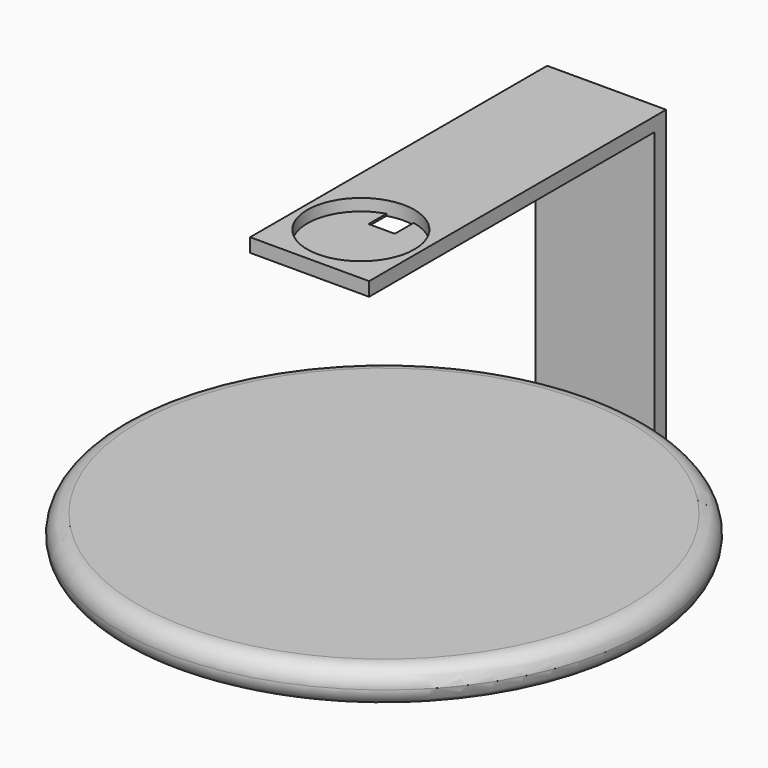
from build123d import *

# Parameters (mm, degrees)
F0_R      = 28.1709911247
F1_DEPTH  = 3.81
F2_R      = 1.90499
F4_DEPTH  = 31.75
F5_W      = 12.7
F5_H      = 1.4726919234
F6_DEPTH  = 38.1
F8_DEPTH  = 12.7
F9_R      = 5.715
F10_DEPTH = 1.27
F12_DEPTH = 25.4


# Not quite as in the source:
# - a fillet or chamfer is up to 0.001 mm smaller than in the source, because OpenCascade refuses the exact size


with BuildPart() as f1:
    # F0 (on Top) → F1 (new body)
    with BuildSketch(Plane.XY):
        Circle(F0_R)
    extrude(amount=F1_DEPTH)

    # F2 (radius 1.905 in the source; OpenCascade refuses exactly that, so slightly less here)
    f2_edges = [f1.edges().sort_by_distance(p)[0] for p in [
        (-28.170991, 0, 3.81),
        (-28.170991, 0, 0),
    ]]
    fillet(f2_edges, radius=F2_R)


with BuildPart() as f4:
    # F3 (on face) → F4 (new body)
    with BuildSketch(Plane(origin=(0, 0, 0), x_dir=(1, 0, 0), z_dir=(0, 0, -1))):
        Polygon((6.35, -28.1780194491), (0, -28.1780194491), (-6.35, -28.1780194491), (-6.35, -29.7020194491), (6.35, -29.7020194491), align=None)
    extrude(amount=-F4_DEPTH)

    # F5 (on face) → F6 (join)
    with BuildSketch(Plane.XZ.offset(-28.1780194491)):
        with Locations((0, 31.0136540383)):
            Rectangle(F5_W, F5_H)
    extrude(amount=F6_DEPTH)

    # F9 (on face) → F10 (cut)
    with BuildSketch(Plane.XY.offset(31.75)):
        with Locations((0, -3.0844647083)):
            Circle(F9_R)
    extrude(amount=-F10_DEPTH, mode=Mode.SUBTRACT)

    # F11 (on face) → F12 (cut)
    with BuildSketch(Plane.XY.offset(30.48)):
        with BuildLine():
            ThreePointArc((1.1540995911, 2.5127916851), (-0.2566010446, 2.6247717471), (-1.6515682438, 2.3866912332))
            Line((-1.6515682438, 2.3866912332), (-1.6515682438, 0))
            Line((-1.6515682438, 0), (1.1540995911, 0))
            Line((1.1540995911, 0), (1.1540995911, 2.5127916851))
        make_face()
    extrude(amount=-F12_DEPTH, mode=Mode.SUBTRACT)


with BuildPart() as f8:
    # F7 (on face) → F8 (new body)
    with BuildSketch(Plane(origin=(-6.35, 0, 0), x_dir=(0, -1, 0), z_dir=(-1, 0, 0))):
        Polygon((-28.1780194491, 1.9405478379), (-28.1780194491, 0), (-25.6668012589, 0), align=None)
    extrude(amount=-F8_DEPTH)


solid = Compound([f1.part, f4.part, f8.part])
